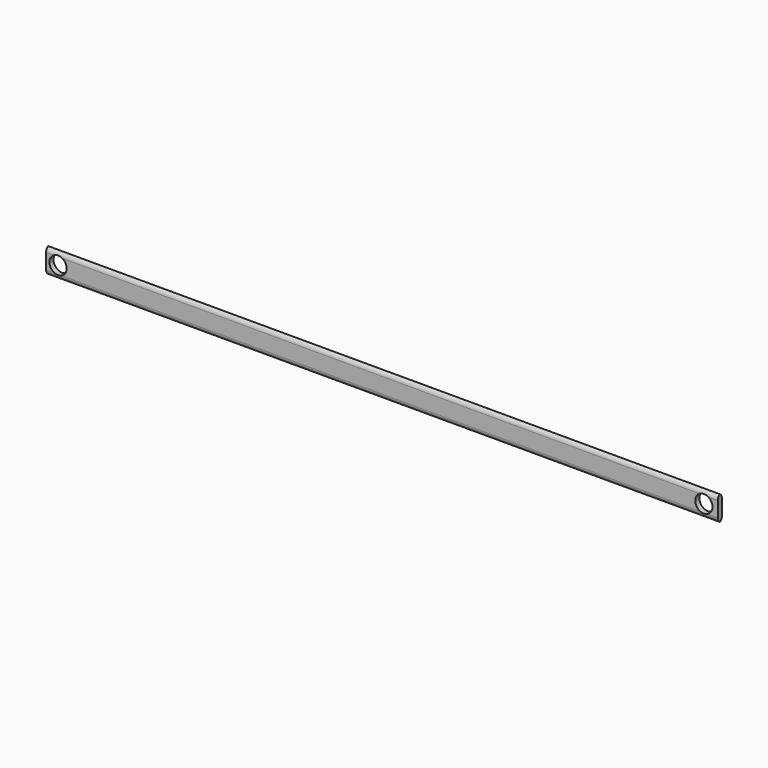
from build123d import *

# Parameters (mm, degrees)
F0_W        = 390
F0_H        = 15
F1_DEPTH    = 3
F2_R        = 5
F3_DEPTH    = 20
F4_T1_DEPTH = 405


# Not quite as in the source:
# - a fillet or chamfer that OpenCascade refuses, or shapes differently, is made with other operations: its cross-section is extruded or revolved along the edge and cut away or added


with BuildPart() as f1:
    # F0 (on Front) → F1 (new body)
    with BuildSketch(Plane.XZ):
        with Locations((-195, 7.5)):
            Rectangle(F0_W, F0_H)
    extrude(amount=F1_DEPTH)

    # F2 (on Front) → F3 (cut)
    with BuildSketch(Plane.XZ):
        with Locations((-383.0693596974, 7.6079843566)):
            Circle(F2_R)
        with Locations((-8.0693596974, 7.6553751715)):
            Circle(F2_R)
    extrude(amount=F3_DEPTH, mode=Mode.SUBTRACT)

    # F4: fillet of radius 3 on 4 edges, made by hand

    # F4_s2 → F4_t1 (cut)
    with BuildSketch(Plane.YZ.offset(-397.5)):
        with BuildLine():
            ThreePointArc((-3, 15), (-0.8786796564, 14.1213203436), (0, 12))
            Line((0, 12), (0, 15))
            Line((0, 15), (-3, 15))
        make_face()
        with BuildLine():
            ThreePointArc((0, 3), (-0.8786796564, 0.8786796564), (-3, 0))
            Line((-3, 0), (0, 0))
            Line((0, 0), (0, 3))
        make_face()
        with BuildLine():
            ThreePointArc((0, 15), (-2.1213203436, 14.1213203436), (-3, 12))
            Line((-3, 12), (-3, 15))
            Line((-3, 15), (0, 15))
        make_face()
        with BuildLine():
            ThreePointArc((-3, 3), (-2.1213203436, 0.8786796564), (0, 0))
            Line((0, 0), (-3, 0))
            Line((-3, 0), (-3, 3))
        make_face()
    extrude(amount=F4_T1_DEPTH, mode=Mode.SUBTRACT)


solid = f1.part
